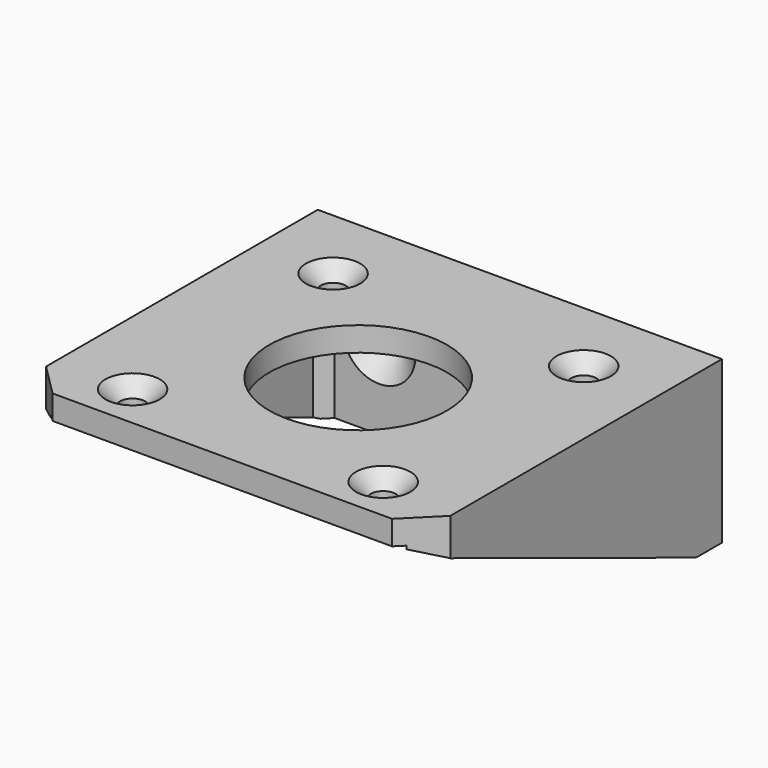
from build123d import *

# Parameters (mm, degrees)
F0_W           = 50
F0_H           = 46
F0_R           = 11
F1_DEPTH       = 20
F2_W           = 44
F2_H           = 43
F3_DEPTH       = 17
F4_SIZE2       = 17
F4_SIZE        = 42
F5_D           = 3.1
F5_CSINK_D     = 6.72
F5_CSINK_ANGLE = 90
F6_T1_DEPTH    = 23.5734639037
F7_SIZE        = 1.5
F9_D           = 4.1
F9_CSINK_D     = 9
F9_CSINK_ANGLE = 90


# Not quite as in the source:
# - a fillet or chamfer that OpenCascade refuses, or shapes differently, is made with other operations: its cross-section is extruded or revolved along the edge and cut away or added


with BuildPart() as f1:
    # F0 (on Top) → F1 (new body)
    with BuildSketch(Plane.XY):
        with Locations((0, 2)):
            Rectangle(F0_W, F0_H)
        Circle(F0_R, mode=Mode.SUBTRACT)
    extrude(amount=-F1_DEPTH)

    # F2 (on face) → F3 (cut, through all)
    with BuildSketch(Plane(origin=(0, 0, -20), x_dir=(1, 0, 0), z_dir=(0, 0, -1))):
        with Locations((0, -0.5)):
            Rectangle(F2_W, F2_H)
    extrude(amount=-F3_DEPTH, mode=Mode.SUBTRACT)

    # F4
    f4_edges = [f1.edges().sort_by_distance(p)[0] for p in [
        (23.5, -21, -20),
        (-23.5, -21, -20),
    ]]
    f4_side = f1.faces().sort_by_distance((-24.320588, 2, -20))[0]
    chamfer(f4_edges, length=F4_SIZE, length2=F4_SIZE2, reference=f4_side)

    # F5 (through all)
    with Locations(Plane.XY):
        with Locations((15.5, 15.5), (-15.5, 15.5), (-15.5, -15.5), (15.5, -15.5)):
            CounterSinkHole(F5_D / 2, F5_CSINK_D / 2, counter_sink_angle=F5_CSINK_ANGLE)

    # F6: chamfer of 4 on 2 edges, made by hand

    # F6_s2 → F6_t1 (cut)
    with BuildSketch(Plane.XY.offset(-13.2867319519)):
        Polygon((-21, -21), (-25, -17), (-25, -21), align=None)
        Polygon((21, -21), (25, -17), (25, -21), align=None)
    extrude(amount=F6_T1_DEPTH, mode=Mode.SUBTRACT)

    # F7
    f7_edges = [f1.edges().sort_by_distance(p)[0] for p in [
        (-22, 22, -11.5),
        (22, 22, -11.5),
    ]]
    chamfer(f7_edges, length=F7_SIZE)

    # F9 (through all)
    with Locations(Plane.XZ.offset(-22)):
        with Locations((15, -10), (-15, -10)):
            CounterSinkHole(F9_D / 2, F9_CSINK_D / 2, counter_sink_angle=F9_CSINK_ANGLE)


solid = f1.part
